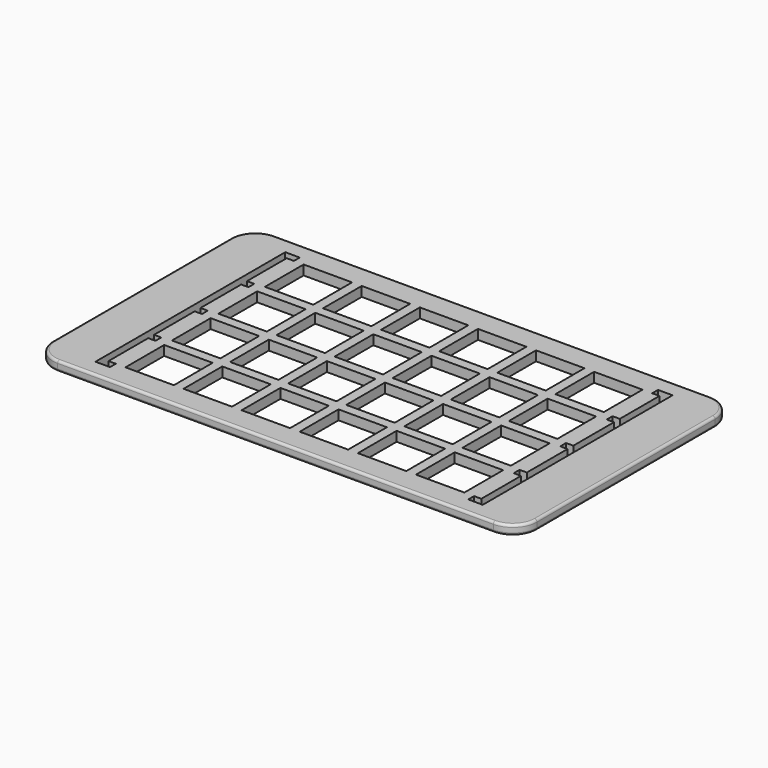
from build123d import *

# Parameters (mm, degrees)
F0_W     = 10
F0_H     = 10
F0_H_2   = 46
F0_W_2   = 1.5
F0_H_3   = 10.5
F0_H_4   = 10.25
F1_DEPTH = 2
F2_R     = 5
F4_R     = 0.5


# Not quite as in the source:
# - two fillets or chamfers of one size are made in one step


with BuildPart() as f1:
    # F0 (on Top) → F1 (new body)
    with BuildSketch(Plane.XY):
        Polygon((-43, 29), (-41, 29), (-41, 34), (-46, 34), (-46, 30.5), (-43, 30.5), align=None)
        Polygon((-41, 34), (-41, 29), (-43, 29), (-43, 18.75), (-43, 17.25), (-43, 6.75), (-43, 5.25), (-43, -5.25), (-43, -6.75), (-43, -17), (-43, -18.5), (-46, -18.5), (-46, -22), (29, -22), (29, -17), (31, -17), (31, -6.75), (31, -5.25), (31, 5.25), (31, 6.75), (31, 17.25), (31, 18.75), (31, 29), (31, 30.5), (34, 30.5), (34, 34), align=None)
        with Locations((-36, -12)):
            Rectangle(F0_W, F0_H, mode=Mode.SUBTRACT)
        with Locations((-24, -12)):
            Rectangle(F0_W, F0_H, mode=Mode.SUBTRACT)
        with Locations((-12, -12)):
            Rectangle(F0_W, F0_H, mode=Mode.SUBTRACT)
        with Locations((-36, 0)):
            Rectangle(F0_W, F0_H, mode=Mode.SUBTRACT)
        with Locations((-24, 0)):
            Rectangle(F0_W, F0_H, mode=Mode.SUBTRACT)
        with Locations((-12, 0)):
            Rectangle(F0_W, F0_H, mode=Mode.SUBTRACT)
        with Locations((0, -12)):
            Rectangle(F0_W, F0_H, mode=Mode.SUBTRACT)
        with Locations((12, -12)):
            Rectangle(F0_W, F0_H, mode=Mode.SUBTRACT)
        with Locations((24, -12)):
            Rectangle(F0_W, F0_H, mode=Mode.SUBTRACT)
        Rectangle(F0_W, F0_H, mode=Mode.SUBTRACT)
        with Locations((12, 0)):
            Rectangle(F0_W, F0_H, mode=Mode.SUBTRACT)
        with Locations((24, 0)):
            Rectangle(F0_W, F0_H, mode=Mode.SUBTRACT)
        with Locations((-36, 12)):
            Rectangle(F0_W, F0_H, mode=Mode.SUBTRACT)
        with Locations((-24, 12)):
            Rectangle(F0_W, F0_H, mode=Mode.SUBTRACT)
        with Locations((-12, 12)):
            Rectangle(F0_W, F0_H, mode=Mode.SUBTRACT)
        with Locations((-36, 24)):
            Rectangle(F0_W, F0_H, mode=Mode.SUBTRACT)
        with Locations((-24, 24)):
            Rectangle(F0_W, F0_H, mode=Mode.SUBTRACT)
        with Locations((-12, 24)):
            Rectangle(F0_W, F0_H, mode=Mode.SUBTRACT)
        with Locations((0, 12)):
            Rectangle(F0_W, F0_H, mode=Mode.SUBTRACT)
        with Locations((12, 12)):
            Rectangle(F0_W, F0_H, mode=Mode.SUBTRACT)
        with Locations((24, 12)):
            Rectangle(F0_W, F0_H, mode=Mode.SUBTRACT)
        with Locations((0, 24)):
            Rectangle(F0_W, F0_H, mode=Mode.SUBTRACT)
        with Locations((12, 24)):
            Rectangle(F0_W, F0_H, mode=Mode.SUBTRACT)
        with Locations((24, 24)):
            Rectangle(F0_W, F0_H, mode=Mode.SUBTRACT)
        Polygon((44, 34), (34, 34), (34, 30.5), (34, 29), (44, 29), align=None)
        with Locations((39, 6)):
            Rectangle(F0_W, F0_H_2)
        Polygon((44, -22), (44, -17), (34, -17), (34, -18.5), (34, -22), align=None)
        Polygon((34, -22), (34, -18.5), (31, -18.5), (31, -17), (29, -17), (29, -22), align=None)
        with Locations((31.75, 0)):
            Rectangle(F0_W_2, F0_H_3)
        with Locations((31.75, 12)):
            Rectangle(F0_W_2, F0_H_3)
        with Locations((-51, 6)):
            Rectangle(F0_W, F0_H_2)
        Polygon((-46, -18.5), (-46, -17), (-56, -17), (-56, -22), (-46, -22), align=None)
        Polygon((-46, 30.5), (-46, 34), (-56, 34), (-56, 29), (-46, 29), align=None)
        with Locations((-43.75, 23.875)):
            Rectangle(F0_W_2, F0_H_4)
        with Locations((-43.75, 12)):
            Rectangle(F0_W_2, F0_H_3)
        with Locations((-43.75, 0)):
            Rectangle(F0_W_2, F0_H_3)
        with Locations((-43.75, -11.875)):
            Rectangle(F0_W_2, F0_H_4)
        with Locations((31.75, 23.875)):
            Rectangle(F0_W_2, F0_H_4)
        with Locations((31.75, -11.875)):
            Rectangle(F0_W_2, F0_H_4)
    extrude(amount=F1_DEPTH)

    # F2
    f2_edges = [f1.edges().sort_by_distance(p)[0] for p in [
        (44, -22, 1),
        (44, 34, 1),
        (-56, 34, 1),
        (-56, -22, 1),
    ]]
    fillet(f2_edges, radius=F2_R)

    # F4
    f4_edges = [f1.edges().sort_by_distance(p)[0] for p in [
        (-6, 34, 2),
        (-6, 34, 0),
        (-51, 34, 1),
        (39, 34, 1),
        (44, 6, 2),
        (44, 29, 1),
        (44, 6, 0),
        (42.535534, 32.535534, 2),
        (-6, -22, 2),
        (42.535534, 32.535534, 0),
        (-6, -22, 0),
        (-56, 6, 2),
        (-54.535534, 32.535534, 2),
        (-56, 6, 0),
        (-56, 29, 1),
        (-54.535534, 32.535534, 0),
        (42.535534, -20.535534, 0),
        (-54.535534, -20.535534, 0),
        (42.535534, -20.535534, 2),
        (-54.535534, -20.535534, 2),
    ]]
    fillet(f4_edges, radius=F4_R)


solid = f1.part
